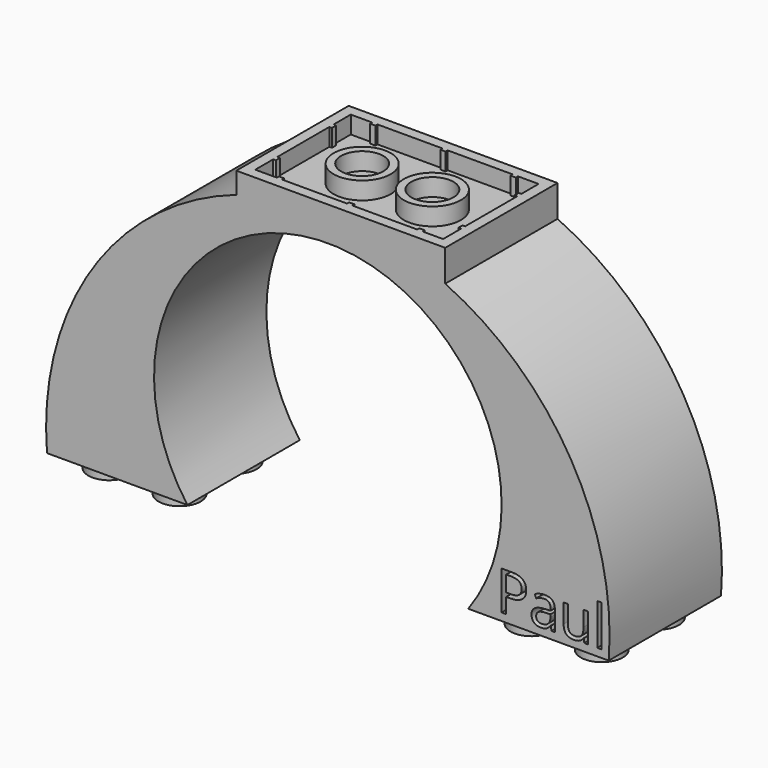
from build123d import *

# Parameters (mm, degrees)
F1_DEPTH      = 16
F2_R          = 2.4
F3_DEPTH      = 1.8
F4_R          = 1.3
F5_DEPTH      = 1.2
F6_R          = 1.3
F7_DEPTH      = 1.2
F9_W          = 23.8
F9_H          = 16
F10_DEPTH     = 3.2
F11_DEPTH     = 0.5
F13_W         = 21.4
F13_H         = 13.6
F14_DEPTH     = 2
F12_R         = 3.255
F12_R_2       = 2.4
F15_DEPTH     = 3.2
F16_W         = 0.6
F16_H         = 0.3
F17_DEPTH     = 3.2
F18_W         = 0.3
F18_H         = 0.6
F19_DEPTH     = 3.2
F20_TEXT_SIZE = 6.1931581715
F21_DEPTH     = 3.2


# Not quite as in the source:
# - Text() gives the source's letters only with a copy of the font that has no kerning and outlines rounded to 1/6400 em; it was checked with that copy


with BuildPart() as f1:
    # F0 (on Front) → F1 (new body)
    with BuildSketch(Plane.XZ):
        with BuildLine():
            ThreePointArc((-17.472484909, -0.1494308526), (-1.472484909, 31.3185100708), (14.527515091, -0.1494308526))
            Line((14.527515091, -0.1494308526), (30.527515091, -0.1494308526))
            ThreePointArc((30.527515091, -0.1494308526), (-1.472484909, 34.5185100708), (-33.472484909, -0.1494308526))
            Line((-33.472484909, -0.1494308526), (-17.472484909, -0.1494308526))
        make_face()
    extrude(amount=F1_DEPTH)

    # F2 (on face) → F3 (join)
    with BuildSketch(Plane(origin=(0, 0, -0.1494308526), x_dir=(1, 0, 0), z_dir=(0, 0, -1))):
        with Locations((-29.522484909, 12.05)):
            Circle(F2_R)
        with Locations((-29.522484909, 4.05)):
            Circle(F2_R)
        with Locations((-21.522484909, 12.05)):
            Circle(F2_R)
        with Locations((-21.522484909, 4.05)):
            Circle(F2_R)
        with Locations((26.577515091, 12.05)):
            Circle(F2_R)
        with Locations((26.577515091, 4.05)):
            Circle(F2_R)
        with Locations((18.577515091, 12.05)):
            Circle(F2_R)
        with Locations((18.577515091, 4.05)):
            Circle(F2_R)
    extrude(amount=F3_DEPTH)

    # F4 (on Top) → F5 (cut)
    with BuildSketch(Plane.XY):
        with Locations((-29.522484909, -4.05)):
            Circle(F4_R)
        with Locations((-29.522484909, -12.05)):
            Circle(F4_R)
        with Locations((-21.522484909, -4.05)):
            Circle(F4_R)
        with Locations((-21.522484909, -12.05)):
            Circle(F4_R)
    extrude(amount=-F5_DEPTH, mode=Mode.SUBTRACT)

    # F6 (on Top) → F7 (cut)
    with BuildSketch(Plane.XY):
        with Locations((18.577515091, -4.05)):
            Circle(F6_R)
        with Locations((18.577515091, -12.05)):
            Circle(F6_R)
        with Locations((26.577515091, -4.05)):
            Circle(F6_R)
        with Locations((26.577515091, -12.05)):
            Circle(F6_R)
    extrude(amount=-F7_DEPTH, mode=Mode.SUBTRACT)

    # F9 (on offset) → F10 (join)
    with BuildSketch(Plane.XY.offset(32)):
        with Locations((0, -8)):
            Rectangle(F9_W, F9_H)
    extrude(amount=F10_DEPTH)

    # F9 (on offset) → F11 (join)
    with BuildSketch(Plane.XY.offset(32)):
        with Locations((0, -8)):
            Rectangle(F9_W, F9_H)
    extrude(amount=-F11_DEPTH)

    # F13 (on face) → F14 (cut)
    with BuildSketch(Plane.XY.offset(35.2)):
        with Locations((0, -8)):
            Rectangle(F13_W, F13_H)
    extrude(amount=-F14_DEPTH, mode=Mode.SUBTRACT)

    # F12 (on face) → F15 (join)
    with BuildSketch(Plane.XY.offset(35.2)):
        with Locations((-4, -7.95)):
            Circle(F12_R)
        with Locations((-4, -7.95)):
            Circle(F12_R_2, mode=Mode.SUBTRACT)
        with Locations((4, -7.95)):
            Circle(F12_R)
        with Locations((4, -7.95)):
            Circle(F12_R_2, mode=Mode.SUBTRACT)
    extrude(amount=-F15_DEPTH)

    # F16 (on face) → F17 (join)
    with BuildSketch(Plane.XY.offset(35.2)):
        with Locations((-7.95, -1.35)):
            Rectangle(F16_W, F16_H)
        with Locations((-7.95, -14.65)):
            Rectangle(F16_W, F16_H)
        with Locations((0.05, -1.35)):
            Rectangle(F16_W, F16_H)
        with Locations((0.05, -14.65)):
            Rectangle(F16_W, F16_H)
        with Locations((8.05, -1.35)):
            Rectangle(F16_W, F16_H)
        with Locations((8.05, -14.65)):
            Rectangle(F16_W, F16_H)
    extrude(amount=-F17_DEPTH)

    # F18 (on face) → F19 (join)
    with BuildSketch(Plane.XY.offset(35.2)):
        with Locations((-10.55, -3.95)):
            Rectangle(F18_W, F18_H)
        with Locations((-10.55, -11.95)):
            Rectangle(F18_W, F18_H)
        with Locations((10.55, -3.95)):
            Rectangle(F18_W, F18_H)
        with Locations((10.55, -11.95)):
            Rectangle(F18_W, F18_H)
    extrude(amount=-F19_DEPTH)

    # F20 (on face) → F21 (cut)
    with BuildSketch(Plane.XZ.offset(16)):
        with Locations((17.724044621, 0.7085538236)):
            Text('Paul', F20_TEXT_SIZE, font='Open Sans', text_align=(TextAlign.LEFT, TextAlign.BOTTOM))
    extrude(amount=-F21_DEPTH, mode=Mode.SUBTRACT)


solid = f1.part
